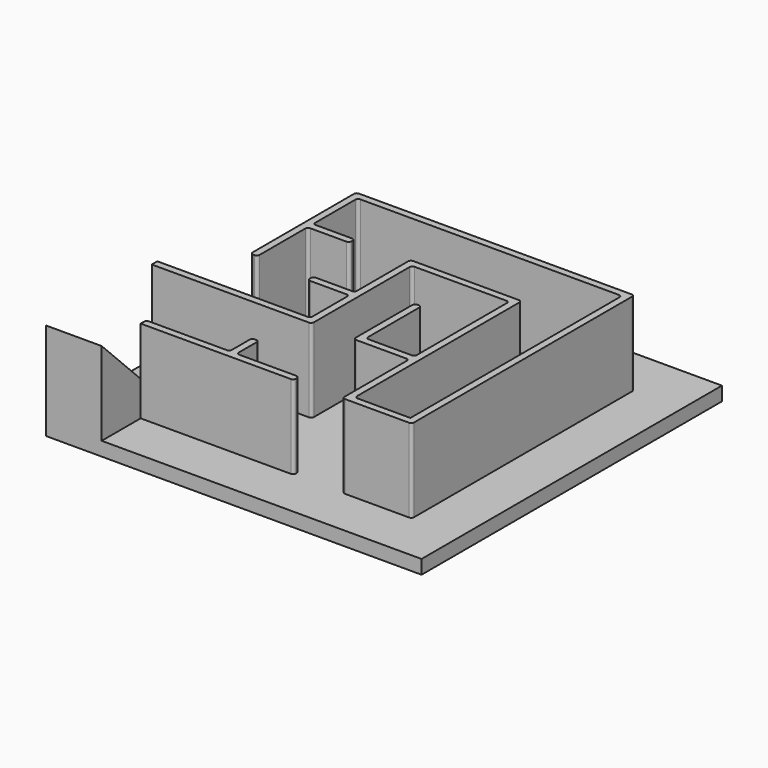
from build123d import *

# Parameters (mm, degrees)
F1_DEPTH = 5
F2_DEPTH = 35
F4_DEPTH = 25
F0_W     = 15
F0_H     = 2.5
F0_W_2   = 2.5
F0_H_2   = 10
F5_DEPTH = 35
F6_R     = 1


# Not quite as in the source:
# - two fillets or chamfers of one size are made in one step


with BuildPart() as f1:
    # F0 (on Top) → F1 (new body)
    with BuildSketch(Plane.XY):
        Polygon((67.5, 67.5), (-67.5, 67.5), (-67.5, -17.5), (-12.5, -17.5), (-12.5, 0), (-27.5, 0), (-27.5, 2.5), (-12.5, 2.5), (-12.5, 25), (-12.5, 27.5), (-10, 27.5), (27.5, 27.5), (27.5, -17.5), (27.5, -20), (27.5, -47.5), (47.5, -47.5), (47.5, 47.5), (-17.5, 47.5), (-17.5, 27.5), (-32.5, 27.5), (-32.5, 25), (-47.5, 25), (-47.5, 2.5), (-50, 2.5), (-50, 50), (50, 50), (50, -50), (25, -50), (25, -20), (5, -20), (5, 7.5), (7.5, 7.5), (7.5, -17.5), (25, -17.5), (25, 25), (-10, 25), (-10, -20), (-67.5, -20), (-67.5, -37.5), (-47.5, -37.5), (-47.5, -47.5), (-17.5, -47.5), (-17.5, -37.5), (-15, -37.5), (-15, -47.5), (7.5, -47.5), (7.5, -50), (-47.5, -50), (-47.5, -67.5), (67.5, -67.5), align=None)
    extrude(amount=F1_DEPTH)

    # F0 (on Top) → F2 (join)
    with BuildSketch(Plane.XY):
        Polygon((-67.5, -67.5), (-47.5, -67.5), (-47.5, -50), (-47.5, -47.5), (-47.5, -37.5), (-67.5, -37.5), align=None)
    extrude(amount=F2_DEPTH)

    # F3 (on face) → F4 (cut)
    with BuildSketch(Plane.YZ.offset(-47.5)):
        Polygon((-37.5, 35), (-67.5, 35), (-37.5, 5), align=None)
    extrude(amount=-F4_DEPTH, mode=Mode.SUBTRACT)

    # F0 (on Top) → F5 (join)
    with BuildSketch(Plane.XY):
        Polygon((27.5, -20), (25, -20), (25, -50), (50, -50), (50, 50), (-50, 50), (-50, 2.5), (-47.5, 2.5), (-47.5, 25), (-47.5, 27.5), (-47.5, 47.5), (-17.5, 47.5), (47.5, 47.5), (47.5, -47.5), (27.5, -47.5), align=None)
        Polygon((-47.5, -47.5), (-47.5, -50), (7.5, -50), (7.5, -47.5), (-15, -47.5), (-17.5, -47.5), align=None)
        Polygon((-12.5, -17.5), (-67.5, -17.5), (-67.5, -20), (-10, -20), (-10, 25), (-12.5, 25), (-12.5, 2.5), (-12.5, 0), align=None)
        with Locations((-20, 1.25)):
            Rectangle(F0_W, F0_H)
        with Locations((-40, 26.25)):
            Rectangle(F0_W, F0_H)
        Polygon((-10, 27.5), (-10, 25), (25, 25), (25, -17.5), (27.5, -17.5), (27.5, 27.5), align=None)
        with Locations((-11.25, 26.25)):
            Rectangle(F0_W_2, F0_H)
        Polygon((25, -20), (25, -17.5), (7.5, -17.5), (7.5, 7.5), (5, 7.5), (5, -20), align=None)
        with Locations((26.25, -18.75)):
            Rectangle(F0_W_2, F0_H)
        with Locations((-16.25, -42.5)):
            Rectangle(F0_W_2, F0_H_2)
    extrude(amount=F5_DEPTH)

    # F6
    f6_edges = [f1.edges().sort_by_distance(p)[0] for p in [
        (7.5, -50, 20),
        (7.5, -47.5, 20),
        (-10, -20, 20),
        (-15, -37.5, 20),
        (5, -20, 20),
        (25, -50, 20),
        (50, -50, 20),
        (27.5, 27.5, 20),
        (50, 50, 20),
        (-47.5, 47.5, 17.5),
        (-27.5, 0, 20),
        (-47.5, 25, 20),
        (-32.5, 25, 20),
        (-32.5, 27.5, 20),
        (-10, 25, 20),
        (7.5, 7.5, 20),
        (-47.5, 2.5, 20),
        (-50, 2.5, 20),
        (-47.5, -47.5, 25),
        (-50, 50, 20),
        (25, -20, 20),
        (-12.5, 2.5, 20),
        (25, -17.5, 20),
        (-12.5, -17.5, 20),
        (27.5, -47.5, 20),
        (-12.5, 27.5, 20),
        (-47.5, 27.5, 17.5),
        (7.5, -17.5, 20),
        (-17.5, -37.5, 20),
        (25, 25, 20),
        (-15, -47.5, 20),
        (-17.5, -47.5, 20),
        (5, 7.5, 20),
        (47.5, 47.5, 20),
        (-27.5, 2.5, 20),
        (-12.5, 0, 20),
    ]]
    fillet(f6_edges, radius=F6_R)


solid = f1.part
